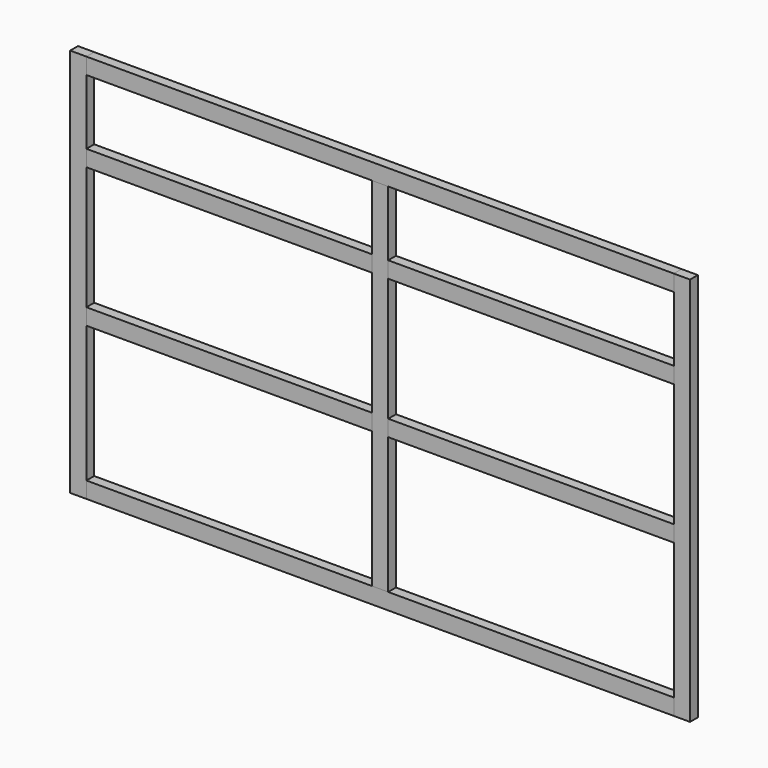
from build123d import *

# Parameters (mm, degrees)
F1_DEPTH = 19.05
F0_W     = 31.75
F0_H     = 241.1844468117
F0_H_2   = 31.75
F0_H_3   = 127.1155531883
F0_H_4   = 266.7
F2_DEPTH = 19.05
F0_W_2   = 558.8


with BuildPart() as f1:
    # F0 (on Front) → F1 (new body)
    with BuildSketch(Plane.XZ):
        Polygon((-504.1488654983, 336.173041563), (-504.1488654983, -425.826958437), (-472.3988654983, -425.826958437), (-472.3988654983, -394.076958437), (-472.3988654983, -127.376958437), (-472.3988654983, -95.626958437), (-472.3988654983, 145.5574883747), (-472.3988654983, 177.3074883747), (-472.3988654983, 304.423041563), (-472.3988654983, 336.173041563), align=None)
    extrude(amount=F1_DEPTH)


with BuildPart() as f1b:
    # F0 (on Front) → F1, piece 2 (new body)
    with BuildSketch(Plane.XZ):
        with Locations((102.2761345017, 24.9652649688)):
            Rectangle(F0_W, F0_H)
        with Locations((102.2761345017, 161.4324883747)):
            Rectangle(F0_W, F0_H_2)
        with Locations((102.2761345017, 240.8652649688)):
            Rectangle(F0_W, F0_H_3)
        with Locations((102.2761345017, -260.726958437)):
            Rectangle(F0_W, F0_H_4)
        with Locations((102.2761345017, -111.501958437)):
            Rectangle(F0_W, F0_H_2)
    extrude(amount=F1_DEPTH)


with BuildPart() as f1c:
    # F0 (on Front) → F1, piece 3 (new body)
    with BuildSketch(Plane.XZ):
        Polygon((676.9511345017, -394.076958437), (676.9511345017, -425.826958437), (708.7011345017, -425.826958437), (708.7011345017, 336.173041563), (676.9511345017, 336.173041563), (676.9511345017, 304.423041563), (676.9511345017, 177.3074883747), (676.9511345017, 145.5574883747), (676.9511345017, -95.626958437), (676.9511345017, -127.376958437), align=None)
    extrude(amount=F1_DEPTH)


with BuildPart() as f2:
    # F0 (on Front) → F2 (new body)
    with BuildSketch(Plane.XZ):
        Polygon((676.9511345017, 336.173041563), (-472.3988654983, 336.173041563), (-472.3988654983, 304.423041563), (86.4011345017, 304.423041563), (118.1511345017, 304.423041563), (676.9511345017, 304.423041563), align=None)
    extrude(amount=F2_DEPTH)


with BuildPart() as f2b:
    # F0 (on Front) → F2, piece 2 (new body)
    with BuildSketch(Plane.XZ):
        with Locations((-192.9988654983, 161.4324883747)):
            Rectangle(F0_W_2, F0_H_2)
    extrude(amount=F2_DEPTH)


with BuildPart() as f2c:
    # F0 (on Front) → F2, piece 3 (new body)
    with BuildSketch(Plane.XZ):
        with Locations((-192.9988654983, -111.501958437)):
            Rectangle(F0_W_2, F0_H_2)
    extrude(amount=F2_DEPTH)


with BuildPart() as f2d:
    # F0 (on Front) → F2, piece 4 (new body)
    with BuildSketch(Plane.XZ):
        Polygon((-472.3988654983, -394.076958437), (-472.3988654983, -425.826958437), (676.9511345017, -425.826958437), (676.9511345017, -394.076958437), (118.1511345017, -394.076958437), (86.4011345017, -394.076958437), align=None)
    extrude(amount=F2_DEPTH)


with BuildPart() as f2e:
    # F0 (on Front) → F2, piece 5 (new body)
    with BuildSketch(Plane.XZ):
        with Locations((397.5511345017, -111.501958437)):
            Rectangle(F0_W_2, F0_H_2)
    extrude(amount=F2_DEPTH)


with BuildPart() as f2f:
    # F0 (on Front) → F2, piece 6 (new body)
    with BuildSketch(Plane.XZ):
        with Locations((397.5511345017, 161.4324883747)):
            Rectangle(F0_W_2, F0_H_2)
    extrude(amount=F2_DEPTH)


solid = Compound([f1.part, f1b.part, f1c.part, f2.part, f2b.part, f2c.part, f2d.part, f2e.part, f2f.part])
